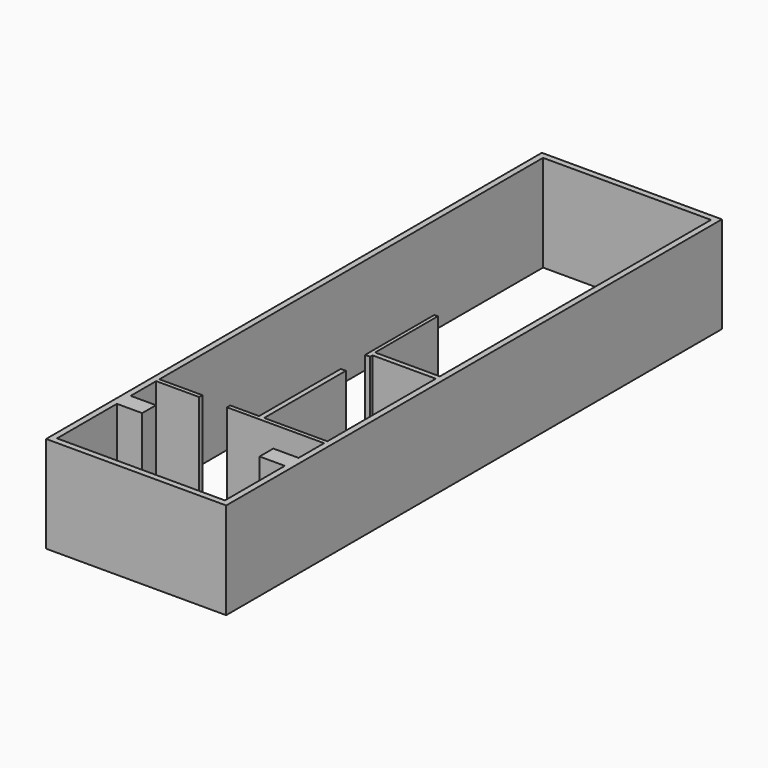
from build123d import *

# Parameters (mm, degrees)
F1_W     = 4521.2
F1_H     = 15557.5
F2_DEPTH = 2425.7


# Not quite as in the source:
# - a feature names something its author has since deleted; it is built from what else it names


with BuildPart() as f2:
    # F1 (on offset) → F2 (new body)
    with BuildSketch(Plane.XY.offset(-406.4)):
        with Locations((2108.2, 5314.95)):
            Rectangle(F1_W, F1_H)
        Polygon((635, 0), (0, 0), (0, 800.1), (1079.5, 800.1), (1079.5, 901.7), (0, 901.7), (0, 12941.3), (4216.4, 12941.3), (4216.4, 4432.3), (2590.8, 4432.3), (2590.8, 6400.8), (2501.9, 6400.8), (2501.9, 4229.1), (2628.9, 4229.1), (2628.9, 4305.3), (4216.4, 4305.3), (4216.4, 901.7), (2628.9, 901.7), (2628.9, 3467.1), (2501.9, 3467.1), (2501.9, 901.7), (1778, 901.7), (1778, 800.1), (4216.4, 800.1), (4216.4, 0), (3581.4, 0), (3581.4, -431.8), (4216.4, -431.8), (4216.4, -2311.4), (0, -2311.4), (0, -431.8), (635, -431.8), align=None, mode=Mode.SUBTRACT)
    extrude(amount=-F2_DEPTH)


solid = f2.part
